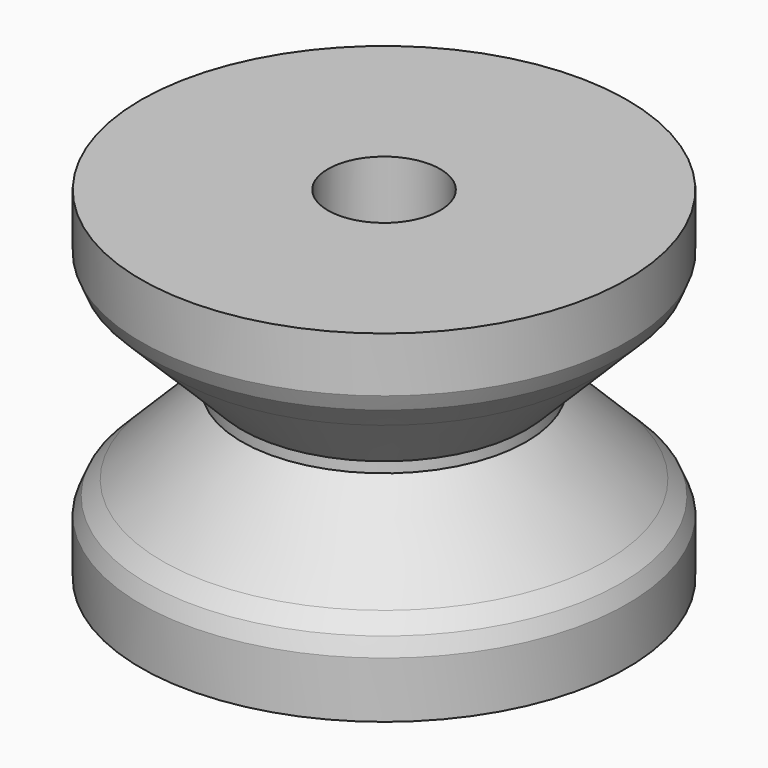
from build123d import *


# Not quite as in the source:
# - a fillet or chamfer that OpenCascade refuses, or shapes differently, is made with other operations: its cross-section is extruded or revolved along the edge and cut away or added


with BuildPart() as f1:
    # F0 (on Front) → F1 (revolve)
    with BuildSketch(Plane.XZ):
        Polygon((2, 1.5050252532), (2, 0), (2, -2), (12, -2), (12, 16.28355698), (2, 16.28355698), (2, 14.28355698), (2, 12.8492424049), (3.8537319575, 10.9955104475), (7.3892658634, 7.4599765415), (7.3892658634, 6.8942911166), (3.1466251763, 2.6516504294), align=None)
    revolve(axis=Axis((15, 0, 2.570889245), (0, 0, 1)))

    # F2: chamfer of 0.5 on 2 edges, made by hand

    # F2_s1 → F2_t2 (revolve, cut)
    with BuildSketch(Plane.XZ):
        Polygon((2, 13.3492424049), (2.3535533906, 12.4956890143), (2, 12.8492424049), align=None)
    revolve(axis=Axis((15, 0, 12.8492424049), (0, 0, 1)), mode=Mode.SUBTRACT)

    # F2_s3 → F2_t4 (revolve, cut)
    with BuildSketch(Plane.XZ):
        Polygon((2.3535533906, 1.8585786438), (2, 1.0050252532), (2, 1.5050252532), align=None)
    revolve(axis=Axis((15, 0, 1.5050252532), (0, 0, 1)), mode=Mode.SUBTRACT)


solid = f1.part
